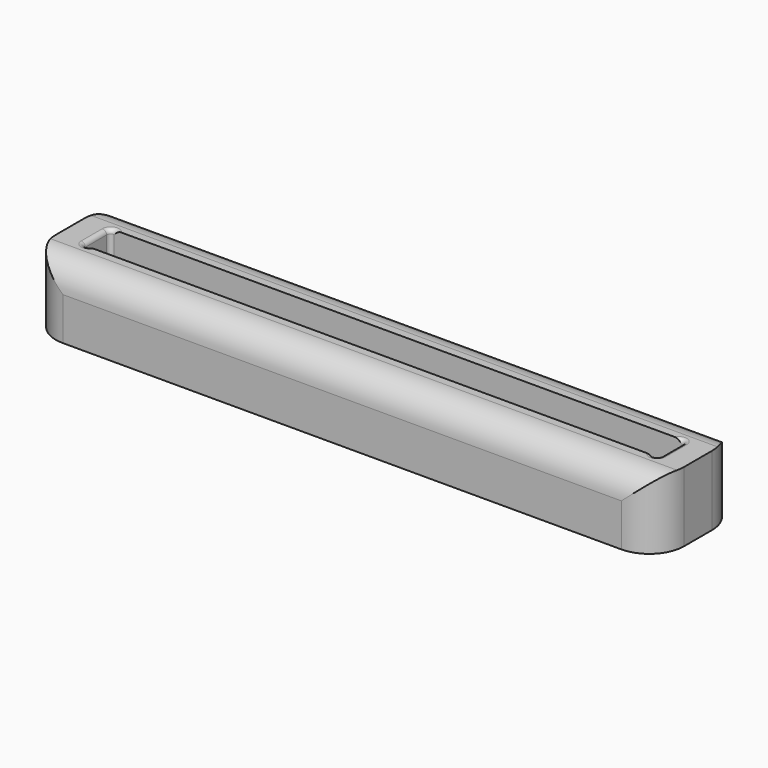
from build123d import *

# Parameters (mm, degrees)
F0_W         = 52.4002
F0_H         = 3.175
F1_DEPTH     = 6.35
F2_T1_DEPTH  = 63.119
F3_T1_DEPTH  = 6.35
F3_T3_DEPTH  = 2.413
F3_T6_ANGLE  = 233.2969892374
F3_T8_ANGLE  = 233.2969892374
F3_T10_ANGLE = 233.2969892374
F3_T12_ANGLE = 233.2969892374


# Not quite as in the source:
# - a fillet or chamfer that OpenCascade refuses, or shapes differently, is made with other operations: its cross-section is extruded or revolved along the edge and cut away or added


with BuildPart() as f1:
    # F0 (on Top) → F1 (new body)
    with BuildSketch(Plane.XY):
        with BuildLine():
            Line((25.4, 4.7625), (-25.4, 4.7625))
            ThreePointArc((-25.4, 4.7625), (-27.6450640303, 3.8325640303), (-28.575, 1.5875))
            Line((-28.575, 1.5875), (-28.575, -1.5875))
            ThreePointArc((-28.575, -1.5875), (-27.6450640303, -3.8325640303), (-25.4, -4.7625))
            Line((-25.4, -4.7625), (25.4, -4.7625))
            ThreePointArc((25.4, -4.7625), (27.6450640303, -3.8325640303), (28.575, -1.5875))
            Line((28.575, -1.5875), (28.575, 1.5875))
            ThreePointArc((28.575, 1.5875), (27.6450640303, 3.8325640303), (25.4, 4.7625))
        make_face()
        Rectangle(F0_W, F0_H, mode=Mode.SUBTRACT)
    extrude(amount=F1_DEPTH)

    # F2: fillet of radius 2.4638 on 2 edges, made by hand

    # F2_s2 → F2_t1 (cut)
    with BuildSketch(Plane.YZ.offset(-31.5595)):
        with BuildLine():
            ThreePointArc((-4.7625, 3.8862), (-4.0408696875, 5.6283696875), (-2.2987, 6.35))
            Line((-2.2987, 6.35), (-4.7625, 6.35))
            Line((-4.7625, 6.35), (-4.7625, 3.8862))
        make_face()
        with BuildLine():
            ThreePointArc((4.7625, 3.8862), (4.0408696875, 5.6283696875), (2.2987, 6.35))
            Line((2.2987, 6.35), (4.7625, 6.35))
            Line((4.7625, 6.35), (4.7625, 3.8862))
        make_face()
    extrude(amount=F2_T1_DEPTH, mode=Mode.SUBTRACT)

    # F3: fillet of radius 0.381 on 6 edges, made by hand

    # F3_s2 → F3_t1 (join)
    with BuildSketch(Plane.XY):
        with BuildLine():
            ThreePointArc((-26.2001, 1.2065), (-26.0885076836, 1.4759076836), (-25.8191, 1.5875))
            Line((-25.8191, 1.5875), (-26.2001, 1.5875))
            Line((-26.2001, 1.5875), (-26.2001, 1.2065))
        make_face()
        with BuildLine():
            ThreePointArc((26.2001, 1.2065), (26.0885076836, 1.4759076836), (25.8191, 1.5875))
            Line((25.8191, 1.5875), (26.2001, 1.5875))
            Line((26.2001, 1.5875), (26.2001, 1.2065))
        make_face()
        with BuildLine():
            ThreePointArc((26.2001, -1.2065), (26.0885076836, -1.4759076836), (25.8191, -1.5875))
            Line((25.8191, -1.5875), (26.2001, -1.5875))
            Line((26.2001, -1.5875), (26.2001, -1.2065))
        make_face()
        with BuildLine():
            ThreePointArc((-25.8191, -1.5875), (-26.0885076836, -1.4759076836), (-26.2001, -1.2065))
            Line((-26.2001, -1.2065), (-26.2001, -1.5875))
            Line((-26.2001, -1.5875), (-25.8191, -1.5875))
        make_face()
    extrude(amount=F3_T1_DEPTH)

    # F3_s4 → F3_t3 (cut)
    with BuildSketch(Plane.XZ.offset(-1.2065)):
        with BuildLine():
            ThreePointArc((-26.2001, 5.969), (-26.3116923164, 6.2384076836), (-26.5811, 6.35))
            Line((-26.5811, 6.35), (-26.2001, 6.35))
            Line((-26.2001, 6.35), (-26.2001, 5.969))
        make_face()
        with BuildLine():
            ThreePointArc((26.2001, 5.969), (26.3116923164, 6.2384076836), (26.5811, 6.35))
            Line((26.5811, 6.35), (26.2001, 6.35))
            Line((26.2001, 6.35), (26.2001, 5.969))
        make_face()
    extrude(amount=F3_T3_DEPTH, mode=Mode.SUBTRACT)

    # F3_s5 → F3_t6 (revolve, cut)
    with BuildSketch(Plane.XZ.offset(-1.2065)):
        with BuildLine():
            ThreePointArc((26.5811, 6.35), (26.3116923164, 6.2384076836), (26.2001, 5.969))
            Line((26.2001, 5.969), (26.2001, 6.35))
            Line((26.2001, 6.35), (26.5811, 6.35))
        make_face()
    revolve(axis=Axis((25.8191, 1.2065, 6.35), (0, 0, 1)), revolution_arc=F3_T6_ANGLE, mode=Mode.SUBTRACT)

    # F3_s7 → F3_t8 (revolve, cut)
    with BuildSketch(Plane.XZ.offset(1.2065)):
        with BuildLine():
            ThreePointArc((26.5811, 6.35), (26.3116923164, 6.2384076836), (26.2001, 5.969))
            Line((26.2001, 5.969), (26.2001, 6.35))
            Line((26.2001, 6.35), (26.5811, 6.35))
        make_face()
    revolve(axis=Axis((25.8191, -1.2065, 6.35), (0, 0, -1)), revolution_arc=F3_T8_ANGLE, mode=Mode.SUBTRACT)

    # F3_s9 → F3_t10 (revolve, cut)
    with BuildSketch(Plane(origin=(-16.0182318513, 11.9409314764, 0), x_dir=(0, 0, 1), z_dir=(-0.8017442393, 0.5976672776, 0))):
        with BuildLine():
            ThreePointArc((6.35, -15.6365356326), (6.2384076836, -15.9059433163), (5.969, -16.0175356326))
            Line((5.969, -16.0175356326), (6.35, -16.0175356326))
            Line((6.35, -16.0175356326), (6.35, -15.6365356326))
        make_face()
    revolve(axis=Axis((-25.8191, -1.2065, 6.35), (0, 0, -1)), revolution_arc=F3_T10_ANGLE, mode=Mode.SUBTRACT)

    # F3_s11 → F3_t12 (revolve, cut)
    with BuildSketch(Plane.XZ.offset(-1.2065)):
        with BuildLine():
            ThreePointArc((-26.5811, 6.35), (-26.3116923164, 6.2384076836), (-26.2001, 5.969))
            Line((-26.2001, 5.969), (-26.2001, 6.35))
            Line((-26.2001, 6.35), (-26.5811, 6.35))
        make_face()
    revolve(axis=Axis((-25.8191, 1.2065, 6.35), (0, 0, -1)), revolution_arc=F3_T12_ANGLE, mode=Mode.SUBTRACT)


solid = f1.part
